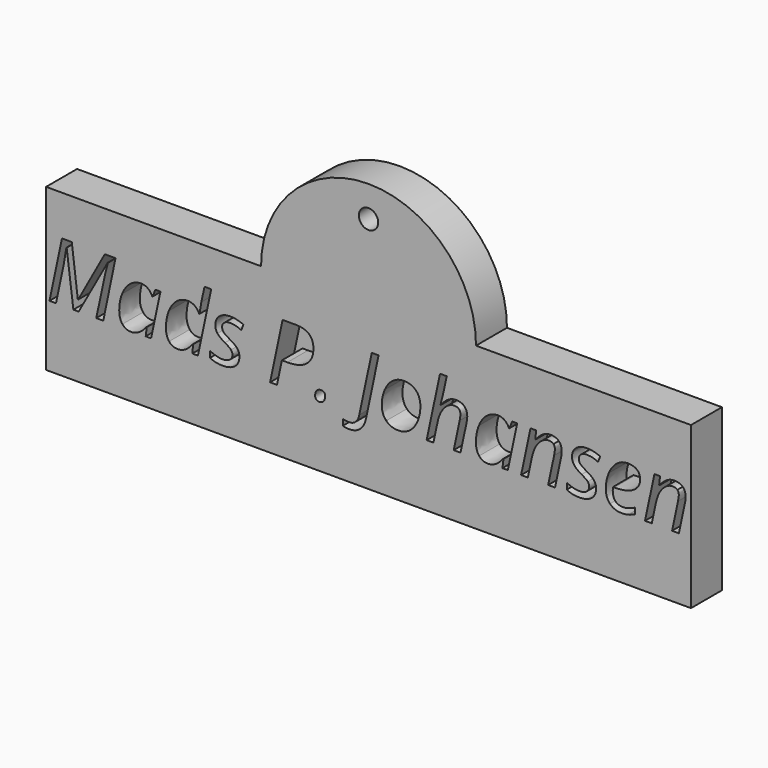
from build123d import *

# Parameters (mm, degrees)
F0_R     = 1.5
F1_DEPTH = 4
F2_R     = 1.5
F3_DEPTH = 2


with BuildPart() as f1:
    # F0 (on Front) → F1 (new body)
    with BuildSketch(Plane.XZ):
        Polygon((-16.667, 12.5), (-50, 12.5), (-50, -12.5), (50, -12.5), (50, 12.5), (16.667, 12.5), (0, 12.5), align=None)
        with BuildLine():
            add(Edge.make_bspline(
                [(-8.1103008935, -2.9097343631), (-8.2795785088, -2.746466604), (-8.2795785088, -2.4279442273)],
                knots=[0, 0, 0, 1, 1, 1], degree=2))
            add(Edge.make_bspline(
                [(-8.2795785088, -2.4279442273), (-8.2795785088, -1.9451524488), (-8.0251612645, -1.6606859237)],
                knots=[0, 0, 0, 1, 1, 1], degree=2))
            add(Edge.make_bspline(
                [(-8.0251612645, -1.6606859237), (-7.7707440202, -1.3762193986), (-7.3280179494, -1.3762193986)],
                knots=[0, 0, 0, 1, 1, 1], degree=2))
            add(Edge.make_bspline(
                [(-7.3280179494, -1.3762193986), (-7.0575744221, -1.3762193986), (-6.8923033775, -1.538485515)],
                knots=[0, 0, 0, 1, 1, 1], degree=2))
            add(Edge.make_bspline(
                [(-6.8923033775, -1.538485515), (-6.727032333, -1.7007516314), (-6.727032333, -2.0332970059)],
                knots=[0, 0, 0, 1, 1, 1], degree=2))
            add(Edge.make_bspline(
                [(-6.727032333, -2.0332970059), (-6.727032333, -2.478026362), (-6.9774430065, -2.7755142421)],
                knots=[0, 0, 0, 1, 1, 1], degree=2))
            add(Edge.make_bspline(
                [(-6.9774430065, -2.7755142421), (-7.22785368, -3.0730021222), (-7.6525501823, -3.0730021222)],
                knots=[0, 0, 0, 1, 1, 1], degree=2))
            add(Edge.make_bspline(
                [(-7.6525501823, -3.0730021222), (-7.9410232782, -3.0730021222), (-8.1103008935, -2.9097343631)],
                knots=[0, 0, 0, 1, 1, 1], degree=2))
        make_face(mode=Mode.SUBTRACT)
        with BuildLine():
            Line((-44.9477142514, -2.8907031519), (-45.7670579751, -2.8907031519))
            Line((-45.7670579751, -2.8907031519), (-46.8067630915, 5.2226026696))
            Line((-46.8067630915, 5.2226026696), (-46.8568452262, 5.2226026696))
            add(Edge.make_bspline(
                [(-46.8568452262, 5.2226026696), (-46.9009175047, 4.7718634573), (-47.0351376257, 3.9865755852)],
                knots=[0, 0, 0, 1, 1, 1], degree=2))
            add(Edge.make_bspline(
                [(-47.0351376257, 3.9865755852), (-47.1693577467, 3.2012877131), (-47.2695220161, 2.7365255031)],
                knots=[0, 0, 0, 1, 1, 1], degree=2))
            Line((-47.2695220161, 2.7365255031), (-48.4594735366, -2.8907031519))
            Line((-48.4594735366, -2.8907031519), (-49.4731359429, -2.8907031519))
            Line((-49.4731359429, -2.8907031519), (-47.5399655435, 6.262307786))
            Line((-47.5399655435, 6.262307786), (-46.0114587924, 6.262307786))
            Line((-46.0114587924, 6.262307786), (-45.079931087, -1.2760551292))
            Line((-45.079931087, -1.2760551292), (-45.0238390961, -1.2760551292))
            Line((-45.0238390961, -1.2760551292), (-40.8970711968, 6.262307786))
            Line((-40.8970711968, 6.262307786), (-39.2323410393, 6.262307786))
            Line((-39.2323410393, 6.262307786), (-41.1294523018, -2.8907031519))
            Line((-41.1294523018, -2.8907031519), (-42.2192395529, -2.8907031519))
            add(Edge.make_bspline(
                [(-42.2192395529, -2.8907031519), (-41.42994511, 0.8033551036), (-41.0102568212, 2.7785944962)],
                knots=[0, 0, 0, 1, 1, 1], degree=2))
            add(Edge.make_bspline(
                [(-41.0102568212, 2.7785944962), (-40.5905685324, 4.7538338888), (-40.4222925598, 5.2346223819)],
                knots=[0, 0, 0, 1, 1, 1], degree=2))
            Line((-40.4222925598, 5.2346223819), (-40.4583516968, 5.2346223819))
            Line((-40.4583516968, 5.2346223819), (-44.9477142514, -2.8907031519))
        make_face(mode=Mode.SUBTRACT)
        with BuildLine():
            add(Edge.make_bspline(
                [(-36.9856564766, 3.4637180989), (-36.2033735326, 4.0967562815), (-35.2698425418, 4.0967562815)],
                knots=[0, 0, 0, 1, 1, 1], degree=2))
            add(Edge.make_bspline(
                [(-35.2698425418, 4.0967562815), (-34.6948996354, 4.0967562815), (-34.2441604231, 3.7862470464)],
                knots=[0, 0, 0, 1, 1, 1], degree=2))
            add(Edge.make_bspline(
                [(-34.2441604231, 3.7862470464), (-33.7934212108, 3.4757378112), (-33.5430105373, 2.8947850487)],
                knots=[0, 0, 0, 1, 1, 1], degree=2))
            Line((-33.5430105373, 2.8947850487), (-33.4728955487, 2.8947850487))
            Line((-33.4728955487, 2.8947850487), (-33.0542089026, 3.9705493021))
            Line((-33.0542089026, 3.9705493021), (-32.2589046035, 3.9705493021))
            Line((-32.2589046035, 3.9705493021), (-33.717296366, -2.8907031519))
            Line((-33.717296366, -2.8907031519), (-34.5506630875, -2.8907031519))
            Line((-34.5506630875, -2.8907031519), (-34.3863936856, -1.5825577935))
            Line((-34.3863936856, -1.5825577935), (-34.4364758203, -1.5825577935))
            add(Edge.make_bspline(
                [(-34.4364758203, -1.5825577935), (-35.5583156376, -3.0169101314), (-36.7983492928, -3.0169101314)],
                knots=[0, 0, 0, 1, 1, 1], degree=2))
            add(Edge.make_bspline(
                [(-36.7983492928, -3.0169101314), (-37.6677751512, -3.0169101314), (-38.1625866421, -2.3968933038)],
                knots=[0, 0, 0, 1, 1, 1], degree=2))
            add(Edge.make_bspline(
                [(-38.1625866421, -2.3968933038), (-38.6573981329, -1.7768764762), (-38.6573981329, -0.6991089374)],
                knots=[0, 0, 0, 1, 1, 1], degree=2))
            add(Edge.make_bspline(
                [(-38.6573981329, -0.6991089374), (-38.6573981329, 0.6030265648), (-38.2126687768, 1.7168532405)],
                knots=[0, 0, 0, 1, 1, 1], degree=2))
            add(Edge.make_bspline(
                [(-38.2126687768, 1.7168532405), (-37.7679394206, 2.8306799163), (-36.9856564766, 3.4637180989)],
                knots=[0, 0, 0, 1, 1, 1], degree=2))
        make_face(mode=Mode.SUBTRACT)
        with BuildLine():
            add(Edge.make_bspline(
                [(-29.7447814416, 3.4757378112), (-28.9775231379, 4.0827332838), (-28.0259625786, 4.0827332838)],
                knots=[0, 0, 0, 1, 1, 1], degree=2))
            add(Edge.make_bspline(
                [(-28.0259625786, 4.0827332838), (-26.8119716335, 4.0827332838), (-26.2670780079, 2.8947850487)],
                knots=[0, 0, 0, 1, 1, 1], degree=2))
            Line((-26.2670780079, 2.8947850487), (-26.2049761609, 2.8947850487))
            add(Edge.make_bspline(
                [(-26.2049761609, 2.8947850487), (-26.0988020353, 3.8643751765), (-25.9225129212, 4.6095973409)],
                knots=[0, 0, 0, 1, 1, 1], degree=2))
            Line((-25.9225129212, 4.6095973409), (-25.4337112865, 6.8512736901))
            Line((-25.4337112865, 6.8512736901), (-24.3960094555, 6.8512736901))
            Line((-24.3960094555, 6.8512736901), (-26.4613966906, -2.8907031519))
            Line((-26.4613966906, -2.8907031519), (-27.330822549, -2.8907031519))
            Line((-27.330822549, -2.8907031519), (-27.1925958572, -1.5825577935))
            Line((-27.1925958572, -1.5825577935), (-27.2426779919, -1.5825577935))
            add(Edge.make_bspline(
                [(-27.2426779919, -1.5825577935), (-27.8757161745, -2.3638390949), (-28.4266196562, -2.6903746131)],
                knots=[0, 0, 0, 1, 1, 1], degree=2))
            add(Edge.make_bspline(
                [(-28.4266196562, -2.6903746131), (-28.9775231379, -3.0169101314), (-29.566489042, -3.0169101314)],
                knots=[0, 0, 0, 1, 1, 1], degree=2))
            add(Edge.make_bspline(
                [(-29.566489042, -3.0169101314), (-30.4359149004, -3.0169101314), (-30.9247165351, -2.4029031599)],
                knots=[0, 0, 0, 1, 1, 1], degree=2))
            add(Edge.make_bspline(
                [(-30.9247165351, -2.4029031599), (-31.4135181698, -1.7888961885), (-31.4135181698, -0.6991089374)],
                knots=[0, 0, 0, 1, 1, 1], degree=2))
            add(Edge.make_bspline(
                [(-31.4135181698, -0.6991089374), (-31.4135181698, 0.6410889872), (-30.9627789575, 1.7549156629)],
                knots=[0, 0, 0, 1, 1, 1], degree=2))
            add(Edge.make_bspline(
                [(-30.9627789575, 1.7549156629), (-30.5120397452, 2.8687423387), (-29.7447814416, 3.4757378112)],
                knots=[0, 0, 0, 1, 1, 1], degree=2))
        make_face(mode=Mode.SUBTRACT)
        with BuildLine():
            add(Edge.make_bspline(
                [(-20.1690772868, -0.245364797), (-20.0248407388, -0.5548723895), (-20.0248407388, -0.9435097548)],
                knots=[0, 0, 0, 1, 1, 1], degree=2))
            add(Edge.make_bspline(
                [(-20.0248407388, -0.9435097548), (-20.0248407388, -1.9211130241), (-20.7169758404, -2.4690115778)],
                knots=[0, 0, 0, 1, 1, 1], degree=2))
            add(Edge.make_bspline(
                [(-20.7169758404, -2.4690115778), (-21.4091109419, -3.0169101314), (-22.6671741656, -3.0169101314)],
                knots=[0, 0, 0, 1, 1, 1], degree=2))
            add(Edge.make_bspline(
                [(-22.6671741656, -3.0169101314), (-23.7249088505, -3.0169101314), (-24.5763051404, -2.5842004876)],
                knots=[0, 0, 0, 1, 1, 1], degree=2))
            Line((-24.5763051404, -2.5842004876), (-24.5763051404, -1.5945775059))
            add(Edge.make_bspline(
                [(-24.5763051404, -1.5945775059), (-24.1375856405, -1.8570078917), (-23.6307544373, -2.0012444396)],
                knots=[0, 0, 0, 1, 1, 1], degree=2))
            add(Edge.make_bspline(
                [(-23.6307544373, -2.0012444396), (-23.1239232341, -2.1454809876), (-22.6912135903, -2.1454809876)],
                knots=[0, 0, 0, 1, 1, 1], degree=2))
            add(Edge.make_bspline(
                [(-22.6912135903, -2.1454809876), (-21.9039224328, -2.1454809876), (-21.5032653552, -1.8329684671)],
                knots=[0, 0, 0, 1, 1, 1], degree=2))
            add(Edge.make_bspline(
                [(-21.5032653552, -1.8329684671), (-21.1026082776, -1.5204559465), (-21.1026082776, -1.0316543118)],
                knots=[0, 0, 0, 1, 1, 1], degree=2))
            add(Edge.make_bspline(
                [(-21.1026082776, -1.0316543118), (-21.1026082776, -0.6750695128), (-21.3209663849, -0.4306686954)],
                knots=[0, 0, 0, 1, 1, 1], degree=2))
            add(Edge.make_bspline(
                [(-21.3209663849, -0.4306686954), (-21.5393244922, -0.1862678781), (-22.266517088, 0.2404319096)],
                knots=[0, 0, 0, 1, 1, 1], degree=2))
            add(Edge.make_bspline(
                [(-22.266517088, 0.2404319096), (-23.0798509556, 0.697180978), (-23.4184061861, 1.1348988353)],
                knots=[0, 0, 0, 1, 1, 1], degree=2))
            add(Edge.make_bspline(
                [(-23.4184061861, 1.1348988353), (-23.7569614167, 1.5726166926), (-23.7569614167, 2.173602309)],
                knots=[0, 0, 0, 1, 1, 1], degree=2))
            add(Edge.make_bspline(
                [(-23.7569614167, 2.173602309), (-23.7569614167, 3.0370183113), (-23.1239232341, 3.5668872964)],
                knots=[0, 0, 0, 1, 1, 1], degree=2))
            add(Edge.make_bspline(
                [(-23.1239232341, 3.5668872964), (-22.4908850515, 4.0967562815), (-21.4591930766, 4.0967562815)],
                knots=[0, 0, 0, 1, 1, 1], degree=2))
            add(Edge.make_bspline(
                [(-21.4591930766, 4.0967562815), (-20.387435394, 4.0967562815), (-19.3918025562, 3.6319940715)],
                knots=[0, 0, 0, 1, 1, 1], degree=2))
            Line((-19.3918025562, 3.6319940715), (-19.7303577868, 2.7745879254))
            Line((-19.7303577868, 2.7745879254), (-20.0809327297, 2.9308441857))
            add(Edge.make_bspline(
                [(-20.0809327297, 2.9308441857), (-20.7139709123, 3.2012877131), (-21.4591930766, 3.2012877131)],
                knots=[0, 0, 0, 1, 1, 1], degree=2))
            add(Edge.make_bspline(
                [(-21.4591930766, 3.2012877131), (-22.0401458392, 3.2012877131), (-22.3726912136, 2.9288409003)],
                knots=[0, 0, 0, 1, 1, 1], degree=2))
            add(Edge.make_bspline(
                [(-22.3726912136, 2.9288409003), (-22.705236588, 2.6563940875), (-22.705236588, 2.2236844437)],
                knots=[0, 0, 0, 1, 1, 1], degree=2))
            add(Edge.make_bspline(
                [(-22.705236588, 2.2236844437), (-22.705236588, 1.8731095008), (-22.4828719099, 1.6226988273)],
                knots=[0, 0, 0, 1, 1, 1], degree=2))
            add(Edge.make_bspline(
                [(-22.4828719099, 1.6226988273), (-22.2605072319, 1.3722881538), (-21.5653672022, 0.9776409324)],
                knots=[0, 0, 0, 1, 1, 1], degree=2))
            add(Edge.make_bspline(
                [(-21.5653672022, 0.9776409324), (-20.8942665972, 0.6030265648), (-20.603790216, 0.3335846801)],
                knots=[0, 0, 0, 1, 1, 1], degree=2))
            add(Edge.make_bspline(
                [(-20.603790216, 0.3335846801), (-20.3133138347, 0.0641427954), (-20.1690772868, -0.245364797)],
                knots=[0, 0, 0, 1, 1, 1], degree=2))
        make_face(mode=Mode.SUBTRACT)
        with BuildLine():
            add(Edge.make_bspline(
                [(-0.3706077968, -2.9287655743), (-0.8654192876, -5.3006554737), (-3.0129412236, -5.3006554737)],
                knots=[0, 0, 0, 1, 1, 1], degree=2))
            add(Edge.make_bspline(
                [(-3.0129412236, -5.3006554737), (-3.6700188309, -5.3006554737), (-3.9705116391, -5.1443992135)],
                knots=[0, 0, 0, 1, 1, 1], degree=2))
            Line((-3.9705116391, -5.1443992135), (-3.9324492167, -4.2248912204))
            add(Edge.make_bspline(
                [(-3.9324492167, -4.2248912204), (-3.5017428583, -4.3490949144), (-3.0249609359, -4.3490949144)],
                knots=[0, 0, 0, 1, 1, 1], degree=2))
            add(Edge.make_bspline(
                [(-3.0249609359, -4.3490949144), (-2.3999358949, -4.3490949144), (-1.9892623903, -3.9584542638)],
                knots=[0, 0, 0, 1, 1, 1], degree=2))
            add(Edge.make_bspline(
                [(-1.9892623903, -3.9584542638), (-1.5785888858, -3.5678136131), (-1.4223326255, -2.8145783072)],
                knots=[0, 0, 0, 1, 1, 1], degree=2))
            Line((-1.4223326255, -2.8145783072), (0.4988180616, 6.262307786))
            Line((0.4988180616, 6.262307786), (1.5645658881, 6.262307786))
            Line((1.5645658881, 6.262307786), (-0.3706077968, -2.9287655743))
        make_face(mode=Mode.SUBTRACT)
        with BuildLine():
            add(Edge.make_bspline(
                [(-9.2371489242, 5.6703369538), (-8.5480187508, 5.0783661217), (-8.5480187508, 3.9024375989)],
                knots=[0, 0, 0, 1, 1, 1], degree=2))
            add(Edge.make_bspline(
                [(-8.5480187508, 3.9024375989), (-8.5480187508, 2.3498914232), (-9.5747025121, 1.5295460568)],
                knots=[0, 0, 0, 1, 1, 1], degree=2))
            add(Edge.make_bspline(
                [(-9.5747025121, 1.5295460568), (-10.6013862735, 0.7092006904), (-12.586642093, 0.7092006904)],
                knots=[0, 0, 0, 1, 1, 1], degree=2))
            Line((-12.586642093, 0.7092006904), (-13.4320285268, 0.7092006904))
            Line((-13.4320285268, 0.7092006904), (-14.2012901158, -2.8907031519))
            Line((-14.2012901158, -2.8907031519), (-15.2650346568, -2.8907031519))
            Line((-15.2650346568, -2.8907031519), (-13.3318642574, 6.262307786))
            Line((-13.3318642574, 6.262307786), (-11.2644737369, 6.262307786))
            add(Edge.make_bspline(
                [(-11.2644737369, 6.262307786), (-9.9262790977, 6.262307786), (-9.2371489242, 5.6703369538)],
                knots=[0, 0, 0, 1, 1, 1], degree=2))
        make_face(mode=Mode.SUBTRACT)
        with BuildLine():
            add(Edge.make_bspline(
                [(3.7551584599, 3.4977739505), (4.5314315477, 4.0586938592), (5.4749789655, 4.0586938592)],
                knots=[0, 0, 0, 1, 1, 1], degree=2))
            add(Edge.make_bspline(
                [(5.4749789655, 4.0586938592), (6.664930486, 4.0586938592), (7.3540606595, 3.3545390453)],
                knots=[0, 0, 0, 1, 1, 1], degree=2))
            add(Edge.make_bspline(
                [(7.3540606595, 3.3545390453), (8.043190833, 2.6503842314), (8.043190833, 1.4163604323)],
                knots=[0, 0, 0, 1, 1, 1], degree=2))
            add(Edge.make_bspline(
                [(8.043190833, 1.4163604323), (8.043190833, 0.2404319096), (7.5924516207, -0.805283063)],
                knots=[0, 0, 0, 1, 1, 1], degree=2))
            add(Edge.make_bspline(
                [(7.5924516207, -0.805283063), (7.1417124083, -1.8509980355), (6.3714491766, -2.4209327284)],
                knots=[0, 0, 0, 1, 1, 1], degree=2))
            add(Edge.make_bspline(
                [(6.3714491766, -2.4209327284), (5.6011859449, -2.9908674213), (4.6315958171, -2.9908674213)],
                knots=[0, 0, 0, 1, 1, 1], degree=2))
            add(Edge.make_bspline(
                [(4.6315958171, -2.9908674213), (3.4296245843, -2.9908674213), (2.746504267, -2.2837076794)],
                knots=[0, 0, 0, 1, 1, 1], degree=2))
            add(Edge.make_bspline(
                [(2.746504267, -2.2837076794), (2.0633839497, -1.5765479374), (2.0633839497, -0.3485339945)],
                knots=[0, 0, 0, 1, 1, 1], degree=2))
            add(Edge.make_bspline(
                [(2.0633839497, -0.3485339945), (2.0633839497, 0.841417526), (2.5211346608, 1.8891357839)],
                knots=[0, 0, 0, 1, 1, 1], degree=2))
            add(Edge.make_bspline(
                [(2.5211346608, 1.8891357839), (2.978885372, 2.9368540419), (3.7551584599, 3.4977739505)],
                knots=[0, 0, 0, 1, 1, 1], degree=2))
        make_face(mode=Mode.SUBTRACT)
        with BuildLine():
            Line((14.259385392, -2.8907031519), (13.2076605633, -2.8907031519))
            Line((13.2076605633, -2.8907031519), (14.135181698, 1.4424031424))
            add(Edge.make_bspline(
                [(14.135181698, 1.4424031424), (14.2473656797, 2.0293657611), (14.2473656797, 2.2857862908)],
                knots=[0, 0, 0, 1, 1, 1], degree=2))
            add(Edge.make_bspline(
                [(14.2473656797, 2.2857862908), (14.2473656797, 3.2133074254), (13.3278576866, 3.2133074254)],
                knots=[0, 0, 0, 1, 1, 1], degree=2))
            add(Edge.make_bspline(
                [(13.3278576866, 3.2133074254), (12.7689410633, 3.2133074254), (12.2400737209, 2.8437012713)],
                knots=[0, 0, 0, 1, 1, 1], degree=2))
            add(Edge.make_bspline(
                [(12.2400737209, 2.8437012713), (11.7112063785, 2.4740951172), (11.3075443728, 1.7699403033)],
                knots=[0, 0, 0, 1, 1, 1], degree=2))
            add(Edge.make_bspline(
                [(11.3075443728, 1.7699403033), (10.9038823671, 1.0657854894), (10.6975439721, 0.0701526516)],
                knots=[0, 0, 0, 1, 1, 1], degree=2))
            Line((10.6975439721, 0.0701526516), (10.0645057895, -2.8907031519))
            Line((10.0645057895, -2.8907031519), (9.0127809608, -2.8907031519))
            Line((9.0127809608, -2.8907031519), (11.0801714812, 6.8512736901))
            Line((11.0801714812, 6.8512736901), (12.1318963099, 6.8512736901))
            add(Edge.make_bspline(
                [(12.1318963099, 6.8512736901), (12.0177090428, 6.3364293454), (11.9145398453, 5.8546392095)],
                knots=[0, 0, 0, 1, 1, 1], degree=2))
            add(Edge.make_bspline(
                [(11.9145398453, 5.8546392095), (11.8113706479, 5.3728490737), (11.7021915942, 4.8750326548)],
                knots=[0, 0, 0, 1, 1, 1], degree=2))
            add(Edge.make_bspline(
                [(11.7021915942, 4.8750326548), (11.5930125406, 4.3772162359), (11.4648022757, 3.8323226103)],
                knots=[0, 0, 0, 1, 1, 1], degree=2))
            add(Edge.make_bspline(
                [(11.4648022757, 3.8323226103), (11.3365920109, 3.2874289848), (11.1663127529, 2.6503842314)],
                knots=[0, 0, 0, 1, 1, 1], degree=2))
            Line((11.1663127529, 2.6503842314), (11.2364277415, 2.6503842314))
            add(Edge.make_bspline(
                [(11.2364277415, 2.6503842314), (11.8253936456, 3.4196458204), (12.3973316239, 3.7511895521)],
                knots=[0, 0, 0, 1, 1, 1], degree=2))
            add(Edge.make_bspline(
                [(12.3973316239, 3.7511895521), (12.9692696021, 4.0827332838), (13.5962979286, 4.0827332838)],
                knots=[0, 0, 0, 1, 1, 1], degree=2))
            add(Edge.make_bspline(
                [(13.5962979286, 4.0827332838), (14.4156416523, 4.0827332838), (14.8633759365, 3.6319940715)],
                knots=[0, 0, 0, 1, 1, 1], degree=2))
            add(Edge.make_bspline(
                [(14.8633759365, 3.6319940715), (15.3111102208, 3.1812548592), (15.3111102208, 2.3559012793)],
                knots=[0, 0, 0, 1, 1, 1], degree=2))
            add(Edge.make_bspline(
                [(15.3111102208, 2.3559012793), (15.3111102208, 1.9672639141), (15.1668736728, 1.3161961629)],
                knots=[0, 0, 0, 1, 1, 1], degree=2))
            add(Edge.make_bspline(
                [(15.1668736728, 1.3161961629), (14.9224728555, 0.108215074), (14.259385392, -2.8907031519)],
                knots=[0, 0, 0, 1, 1, 1], degree=2))
        make_face(mode=Mode.SUBTRACT)
        with BuildLine():
            add(Edge.make_bspline(
                [(18.3290596578, 3.4637180989), (19.1113426019, 4.0967562815), (20.0448735927, 4.0967562815)],
                knots=[0, 0, 0, 1, 1, 1], degree=2))
            add(Edge.make_bspline(
                [(20.0448735927, 4.0967562815), (20.6198164991, 4.0967562815), (21.0705557114, 3.7862470464)],
                knots=[0, 0, 0, 1, 1, 1], degree=2))
            add(Edge.make_bspline(
                [(21.0705557114, 3.7862470464), (21.5212949237, 3.4757378112), (21.7717055972, 2.8947850487)],
                knots=[0, 0, 0, 1, 1, 1], degree=2))
            Line((21.7717055972, 2.8947850487), (21.8418205858, 2.8947850487))
            Line((21.8418205858, 2.8947850487), (22.2605072319, 3.9705493021))
            Line((22.2605072319, 3.9705493021), (23.0558115309, 3.9705493021))
            Line((23.0558115309, 3.9705493021), (21.5974197684, -2.8907031519))
            Line((21.5974197684, -2.8907031519), (20.764053047, -2.8907031519))
            Line((20.764053047, -2.8907031519), (20.9283224488, -1.5825577935))
            Line((20.9283224488, -1.5825577935), (20.8782403141, -1.5825577935))
            add(Edge.make_bspline(
                [(20.8782403141, -1.5825577935), (19.7564004968, -3.0169101314), (18.5163668416, -3.0169101314)],
                knots=[0, 0, 0, 1, 1, 1], degree=2))
            add(Edge.make_bspline(
                [(18.5163668416, -3.0169101314), (17.6469409832, -3.0169101314), (17.1521294924, -2.3968933038)],
                knots=[0, 0, 0, 1, 1, 1], degree=2))
            add(Edge.make_bspline(
                [(17.1521294924, -2.3968933038), (16.6573180015, -1.7768764762), (16.6573180015, -0.6991089374)],
                knots=[0, 0, 0, 1, 1, 1], degree=2))
            add(Edge.make_bspline(
                [(16.6573180015, -0.6991089374), (16.6573180015, 0.6030265648), (17.1020473577, 1.7168532405)],
                knots=[0, 0, 0, 1, 1, 1], degree=2))
            add(Edge.make_bspline(
                [(17.1020473577, 1.7168532405), (17.5467767138, 2.8306799163), (18.3290596578, 3.4637180989)],
                knots=[0, 0, 0, 1, 1, 1], degree=2))
        make_face(mode=Mode.SUBTRACT)
        with BuildLine():
            Line((28.9154212909, -2.8907031519), (27.8516767499, -2.8907031519))
            Line((27.8516767499, -2.8907031519), (28.7791978845, 1.4424031424))
            add(Edge.make_bspline(
                [(28.7791978845, 1.4424031424), (28.9034015786, 2.0934708935), (28.9034015786, 2.343881567)],
                knots=[0, 0, 0, 1, 1, 1], degree=2))
            add(Edge.make_bspline(
                [(28.9034015786, 2.343881567), (28.9034015786, 2.7365255031), (28.6810369005, 2.9749164642)],
                knots=[0, 0, 0, 1, 1, 1], degree=2))
            add(Edge.make_bspline(
                [(28.6810369005, 2.9749164642), (28.4586722224, 3.2133074254), (27.9718738732, 3.2133074254)],
                knots=[0, 0, 0, 1, 1, 1], degree=2))
            add(Edge.make_bspline(
                [(27.9718738732, 3.2133074254), (27.4129572499, 3.2133074254), (26.8840899074, 2.8376914152)],
                knots=[0, 0, 0, 1, 1, 1], degree=2))
            add(Edge.make_bspline(
                [(26.8840899074, 2.8376914152), (26.355222565, 2.4620754049), (25.9515605593, 1.7669353753)],
                knots=[0, 0, 0, 1, 1, 1], degree=2))
            add(Edge.make_bspline(
                [(25.9515605593, 1.7669353753), (25.5478985536, 1.0717953456), (25.3415601587, 0.0821723639)],
                knots=[0, 0, 0, 1, 1, 1], degree=2))
            Line((25.3415601587, 0.0821723639), (24.708521976, -2.8907031519))
            Line((24.708521976, -2.8907031519), (23.6567971473, -2.8907031519))
            Line((23.6567971473, -2.8907031519), (25.1232020514, 3.9705493021))
            Line((25.1232020514, 3.9705493021), (25.9926279098, 3.9705493021))
            Line((25.9926279098, 3.9705493021), (25.854401218, 2.7004663661))
            Line((25.854401218, 2.7004663661), (25.9185063504, 2.7004663661))
            add(Edge.make_bspline(
                [(25.9185063504, 2.7004663661), (26.5194919668, 3.4637180989), (27.0794102328, 3.7802371902)],
                knots=[0, 0, 0, 1, 1, 1], degree=2))
            add(Edge.make_bspline(
                [(27.0794102328, 3.7802371902), (27.6393284987, 4.0967562815), (28.2403141151, 4.0967562815)],
                knots=[0, 0, 0, 1, 1, 1], degree=2))
            add(Edge.make_bspline(
                [(28.2403141151, 4.0967562815), (29.0356184142, 4.0967562815), (29.4953724108, 3.6610417096)],
                knots=[0, 0, 0, 1, 1, 1], degree=2))
            add(Edge.make_bspline(
                [(29.4953724108, 3.6610417096), (29.9551264073, 3.2253271377), (29.9551264073, 2.4440458364)],
                knots=[0, 0, 0, 1, 1, 1], degree=2))
            add(Edge.make_bspline(
                [(29.9551264073, 2.4440458364), (29.9551264073, 1.9492343456), (29.8108898594, 1.3161961629)],
                knots=[0, 0, 0, 1, 1, 1], degree=2))
            Line((29.8108898594, 1.3161961629), (28.9154212909, -2.8907031519))
        make_face(mode=Mode.SUBTRACT)
        with BuildLine():
            add(Edge.make_bspline(
                [(35.1456388477, -0.245364797), (35.2898753956, -0.5548723895), (35.2898753956, -0.9435097548)],
                knots=[0, 0, 0, 1, 1, 1], degree=2))
            add(Edge.make_bspline(
                [(35.2898753956, -0.9435097548), (35.2898753956, -1.9211130241), (34.5977402941, -2.4690115778)],
                knots=[0, 0, 0, 1, 1, 1], degree=2))
            add(Edge.make_bspline(
                [(34.5977402941, -2.4690115778), (33.9056051925, -3.0169101314), (32.6475419688, -3.0169101314)],
                knots=[0, 0, 0, 1, 1, 1], degree=2))
            add(Edge.make_bspline(
                [(32.6475419688, -3.0169101314), (31.5898072839, -3.0169101314), (30.738410994, -2.5842004876)],
                knots=[0, 0, 0, 1, 1, 1], degree=2))
            Line((30.738410994, -2.5842004876), (30.738410994, -1.5945775059))
            add(Edge.make_bspline(
                [(30.738410994, -1.5945775059), (31.177130494, -1.8570078917), (31.6839616972, -2.0012444396)],
                knots=[0, 0, 0, 1, 1, 1], degree=2))
            add(Edge.make_bspline(
                [(31.6839616972, -2.0012444396), (32.1907929004, -2.1454809876), (32.6235025442, -2.1454809876)],
                knots=[0, 0, 0, 1, 1, 1], degree=2))
            add(Edge.make_bspline(
                [(32.6235025442, -2.1454809876), (33.4107937017, -2.1454809876), (33.8114507793, -1.8329684671)],
                knots=[0, 0, 0, 1, 1, 1], degree=2))
            add(Edge.make_bspline(
                [(33.8114507793, -1.8329684671), (34.2121078569, -1.5204559465), (34.2121078569, -1.0316543118)],
                knots=[0, 0, 0, 1, 1, 1], degree=2))
            add(Edge.make_bspline(
                [(34.2121078569, -1.0316543118), (34.2121078569, -0.6750695128), (33.9937497496, -0.4306686954)],
                knots=[0, 0, 0, 1, 1, 1], degree=2))
            add(Edge.make_bspline(
                [(33.9937497496, -0.4306686954), (33.7753916423, -0.1862678781), (33.0481990464, 0.2404319096)],
                knots=[0, 0, 0, 1, 1, 1], degree=2))
            add(Edge.make_bspline(
                [(33.0481990464, 0.2404319096), (32.2348651789, 0.697180978), (31.8963099483, 1.1348988353)],
                knots=[0, 0, 0, 1, 1, 1], degree=2))
            add(Edge.make_bspline(
                [(31.8963099483, 1.1348988353), (31.5577547177, 1.5726166926), (31.5577547177, 2.173602309)],
                knots=[0, 0, 0, 1, 1, 1], degree=2))
            add(Edge.make_bspline(
                [(31.5577547177, 2.173602309), (31.5577547177, 3.0370183113), (32.1907929004, 3.5668872964)],
                knots=[0, 0, 0, 1, 1, 1], degree=2))
            add(Edge.make_bspline(
                [(32.1907929004, 3.5668872964), (32.823831083, 4.0967562815), (33.8555230578, 4.0967562815)],
                knots=[0, 0, 0, 1, 1, 1], degree=2))
            add(Edge.make_bspline(
                [(33.8555230578, 4.0967562815), (34.9272807404, 4.0967562815), (35.9229135783, 3.6319940715)],
                knots=[0, 0, 0, 1, 1, 1], degree=2))
            Line((35.9229135783, 3.6319940715), (35.5843583477, 2.7745879254))
            Line((35.5843583477, 2.7745879254), (35.2337834048, 2.9308441857))
            add(Edge.make_bspline(
                [(35.2337834048, 2.9308441857), (34.6007452222, 3.2012877131), (33.8555230578, 3.2012877131)],
                knots=[0, 0, 0, 1, 1, 1], degree=2))
            add(Edge.make_bspline(
                [(33.8555230578, 3.2012877131), (33.2745702953, 3.2012877131), (32.9420249209, 2.9288409003)],
                knots=[0, 0, 0, 1, 1, 1], degree=2))
            add(Edge.make_bspline(
                [(32.9420249209, 2.9288409003), (32.6094795465, 2.6563940875), (32.6094795465, 2.2236844437)],
                knots=[0, 0, 0, 1, 1, 1], degree=2))
            add(Edge.make_bspline(
                [(32.6094795465, 2.2236844437), (32.6094795465, 1.8731095008), (32.8318442245, 1.6226988273)],
                knots=[0, 0, 0, 1, 1, 1], degree=2))
            add(Edge.make_bspline(
                [(32.8318442245, 1.6226988273), (33.0542089026, 1.3722881538), (33.7493489322, 0.9776409324)],
                knots=[0, 0, 0, 1, 1, 1], degree=2))
            add(Edge.make_bspline(
                [(33.7493489322, 0.9776409324), (34.4204495372, 0.6030265648), (34.7109259185, 0.3335846801)],
                knots=[0, 0, 0, 1, 1, 1], degree=2))
            add(Edge.make_bspline(
                [(34.7109259185, 0.3335846801), (35.0014022998, 0.0641427954), (35.1456388477, -0.245364797)],
                knots=[0, 0, 0, 1, 1, 1], degree=2))
        make_face(mode=Mode.SUBTRACT)
        with BuildLine():
            add(Edge.make_bspline(
                [(40.2540165872, -2.906729435), (39.8032773749, -3.0169101314), (39.2603870347, -3.0169101314)],
                knots=[0, 0, 0, 1, 1, 1], degree=2))
            add(Edge.make_bspline(
                [(39.2603870347, -3.0169101314), (38.1084979366, -3.0169101314), (37.4504186866, -2.3337898141)],
                knots=[0, 0, 0, 1, 1, 1], degree=2))
            add(Edge.make_bspline(
                [(37.4504186866, -2.3337898141), (36.7923394367, -1.6506694967), (36.7923394367, -0.4426884078)],
                knots=[0, 0, 0, 1, 1, 1], degree=2))
            add(Edge.make_bspline(
                [(36.7923394367, -0.4426884078), (36.7923394367, 0.733240115), (37.2591049321, 1.8140125819)],
                knots=[0, 0, 0, 1, 1, 1], degree=2))
            add(Edge.make_bspline(
                [(37.2591049321, 1.8140125819), (37.7258704275, 2.8947850487), (38.4961336592, 3.4957706651)],
                knots=[0, 0, 0, 1, 1, 1], degree=2))
            add(Edge.make_bspline(
                [(38.4961336592, 3.4957706651), (39.2663968909, 4.0967562815), (40.1919147402, 4.0967562815)],
                knots=[0, 0, 0, 1, 1, 1], degree=2))
            add(Edge.make_bspline(
                [(40.1919147402, 4.0967562815), (41.1494851557, 4.0967562815), (41.6322769342, 3.6800729208)],
                knots=[0, 0, 0, 1, 1, 1], degree=2))
            add(Edge.make_bspline(
                [(41.6322769342, 3.6800729208), (42.1150687127, 3.2633895601), (42.1150687127, 2.5181673958)],
                knots=[0, 0, 0, 1, 1, 1], degree=2))
            add(Edge.make_bspline(
                [(42.1150687127, 2.5181673958), (42.1150687127, 1.3923210077), (41.0753635963, 0.7502680408)],
                knots=[0, 0, 0, 1, 1, 1], degree=2))
            add(Edge.make_bspline(
                [(41.0753635963, 0.7502680408), (40.0356584799, 0.108215074), (38.1004847951, 0.108215074)],
                knots=[0, 0, 0, 1, 1, 1], degree=2))
            Line((38.1004847951, 0.108215074), (37.8941464001, 0.108215074))
            Line((37.8941464001, 0.108215074), (37.8701069754, -0.3926062731))
            add(Edge.make_bspline(
                [(37.8701069754, -0.3926062731), (37.8701069754, -1.2119499968), (38.2547377699, -1.672705636)],
                knots=[0, 0, 0, 1, 1, 1], degree=2))
            add(Edge.make_bspline(
                [(38.2547377699, -1.672705636), (38.6393685644, -2.1334612753), (39.4466925758, -2.1334612753)],
                knots=[0, 0, 0, 1, 1, 1], degree=2))
            add(Edge.make_bspline(
                [(39.4466925758, -2.1334612753), (39.8413397973, -2.1334612753), (40.258023158, -2.0202756508)],
                knots=[0, 0, 0, 1, 1, 1], degree=2))
            add(Edge.make_bspline(
                [(40.258023158, -2.0202756508), (40.6747065187, -1.9070900264), (41.2937217036, -1.6065972182)],
                knots=[0, 0, 0, 1, 1, 1], degree=2))
            Line((41.2937217036, -1.6065972182), (41.2937217036, -2.5220986405))
            add(Edge.make_bspline(
                [(41.2937217036, -2.5220986405), (40.7047557995, -2.7965487387), (40.2540165872, -2.906729435)],
                knots=[0, 0, 0, 1, 1, 1], degree=2))
        make_face(mode=Mode.SUBTRACT)
        with BuildLine():
            Line((48.1289314476, -2.8907031519), (47.0651869065, -2.8907031519))
            Line((47.0651869065, -2.8907031519), (47.9927080412, 1.4424031424))
            add(Edge.make_bspline(
                [(47.9927080412, 1.4424031424), (48.1169117352, 2.0934708935), (48.1169117352, 2.343881567)],
                knots=[0, 0, 0, 1, 1, 1], degree=2))
            add(Edge.make_bspline(
                [(48.1169117352, 2.343881567), (48.1169117352, 2.7365255031), (47.8945470572, 2.9749164642)],
                knots=[0, 0, 0, 1, 1, 1], degree=2))
            add(Edge.make_bspline(
                [(47.8945470572, 2.9749164642), (47.6721823791, 3.2133074254), (47.1853840298, 3.2133074254)],
                knots=[0, 0, 0, 1, 1, 1], degree=2))
            add(Edge.make_bspline(
                [(47.1853840298, 3.2133074254), (46.6264674065, 3.2133074254), (46.0976000641, 2.8376914152)],
                knots=[0, 0, 0, 1, 1, 1], degree=2))
            add(Edge.make_bspline(
                [(46.0976000641, 2.8376914152), (45.5687327217, 2.4620754049), (45.165070716, 1.7669353753)],
                knots=[0, 0, 0, 1, 1, 1], degree=2))
            add(Edge.make_bspline(
                [(45.165070716, 1.7669353753), (44.7614087103, 1.0717953456), (44.5550703153, 0.0821723639)],
                knots=[0, 0, 0, 1, 1, 1], degree=2))
            Line((44.5550703153, 0.0821723639), (43.9220321327, -2.8907031519))
            Line((43.9220321327, -2.8907031519), (42.870307304, -2.8907031519))
            Line((42.870307304, -2.8907031519), (44.336712208, 3.9705493021))
            Line((44.336712208, 3.9705493021), (45.2061380664, 3.9705493021))
            Line((45.2061380664, 3.9705493021), (45.0679113747, 2.7004663661))
            Line((45.0679113747, 2.7004663661), (45.1320165071, 2.7004663661))
            add(Edge.make_bspline(
                [(45.1320165071, 2.7004663661), (45.7330021235, 3.4637180989), (46.2929203894, 3.7802371902)],
                knots=[0, 0, 0, 1, 1, 1], degree=2))
            add(Edge.make_bspline(
                [(46.2929203894, 3.7802371902), (46.8528386554, 4.0967562815), (47.4538242718, 4.0967562815)],
                knots=[0, 0, 0, 1, 1, 1], degree=2))
            add(Edge.make_bspline(
                [(47.4538242718, 4.0967562815), (48.2491285709, 4.0967562815), (48.7088825674, 3.6610417096)],
                knots=[0, 0, 0, 1, 1, 1], degree=2))
            add(Edge.make_bspline(
                [(48.7088825674, 3.6610417096), (49.168636564, 3.2253271377), (49.168636564, 2.4440458364)],
                knots=[0, 0, 0, 1, 1, 1], degree=2))
            add(Edge.make_bspline(
                [(49.168636564, 2.4440458364), (49.168636564, 1.9492343456), (49.024400016, 1.3161961629)],
                knots=[0, 0, 0, 1, 1, 1], degree=2))
            Line((49.024400016, 1.3161961629), (48.1289314476, -2.8907031519))
        make_face(mode=Mode.SUBTRACT)
        with BuildLine():
            ThreePointArc((16.667, 12.5), (0, 29.167), (-16.667, 12.5))
            Line((-16.667, 12.5), (0, 12.5))
            Line((0, 12.5), (16.667, 12.5))
        make_face()
        with Locations((0, 24.3615116924)):
            Circle(F0_R, mode=Mode.SUBTRACT)
    extrude(amount=F1_DEPTH)

    # F2 (on face) → F3 (join)
    with BuildSketch(Plane(origin=(0, 0, 0), x_dir=(-1, 0, 0), z_dir=(0, 1, 0))):
        with BuildLine():
            ThreePointArc((16.667, 12.5), (0, 29.167), (-16.667, 12.5))
            Line((-16.667, 12.5), (-50, 12.5))
            Line((-50, 12.5), (-50, -12.5))
            Line((-50, -12.5), (50, -12.5))
            Line((50, -12.5), (50, 12.5))
            Line((50, 12.5), (16.667, 12.5))
        make_face()
        with BuildLine():
            Line((-47.9927080412, 1.4424031424), (-47.0651869065, -2.8907031519))
            Line((-47.0651869065, -2.8907031519), (-48.1289314476, -2.8907031519))
            Line((-48.1289314476, -2.8907031519), (-49.024400016, 1.3161961629))
            add(Edge.make_bspline(
                [(-45.1320165071, 2.7004663661), (-45.7330021235, 3.4637180989), (-46.8528386554, 4.0967562815), (-48.2491285709, 4.0967562815), (-49.168636564, 3.2253271377), (-49.168636564, 1.9492343456), (-49.024400016, 1.3161961629)],
                knots=[0, 0, 0, 1, 2, 3.3233333333, 4.6466666667, 5.4847777778, 5.4847777778, 5.4847777778], degree=2))
            Line((-45.1320165071, 2.7004663661), (-45.0679113747, 2.7004663661))
            Line((-45.0679113747, 2.7004663661), (-45.2061380664, 3.9705493021))
            Line((-45.2061380664, 3.9705493021), (-44.336712208, 3.9705493021))
            Line((-44.336712208, 3.9705493021), (-42.870307304, -2.8907031519))
            Line((-42.870307304, -2.8907031519), (-43.9220321327, -2.8907031519))
            Line((-43.9220321327, -2.8907031519), (-44.5550703153, 0.0821723639))
            add(Edge.make_bspline(
                [(-47.9927080412, 1.4424031424), (-48.1169117352, 2.0934708935), (-48.1169117352, 2.7365255031), (-47.6721823791, 3.2133074254), (-46.6264674065, 3.2133074254), (-45.5687327217, 2.4620754049), (-44.7614087103, 1.0717953456), (-44.5550703153, 0.0821723639)],
                knots=[0, 0, 0, 1, 2.568, 4.136, 5.9362962963, 7.7365925926, 9.5368888889, 9.5368888889, 9.5368888889], degree=2))
        make_face(mode=Mode.SUBTRACT)
        with BuildLine():
            Line((-37.8701069754, -0.3926062731), (-37.8941464001, 0.108215074))
            Line((-37.8941464001, 0.108215074), (-38.1004847951, 0.108215074))
            add(Edge.make_bspline(
                [(-41.2937217036, -2.5220986405), (-40.7047557995, -2.7965487387), (-39.8032773749, -3.0169101314), (-38.1084979366, -3.0169101314), (-36.7923394367, -1.6506694967), (-36.7923394367, 0.733240115), (-37.7258704275, 2.8947850487), (-39.2663968909, 4.0967562815), (-41.1494851557, 4.0967562815), (-42.1150687127, 3.2633895601), (-42.1150687127, 1.3923210077), (-40.0356584799, 0.108215074), (-38.1004847951, 0.108215074)],
                knots=[0, 0, 0, 1, 2, 4.1217712177, 6.2435424354, 8.3090145827, 10.3744867299, 12.4399588772, 14.5769625274, 16.7139661776, 19.9424501868, 23.1709341959, 23.1709341959, 23.1709341959], degree=2))
            Line((-41.2937217036, -2.5220986405), (-41.2937217036, -1.6065972182))
            add(Edge.make_bspline(
                [(-37.8701069754, -0.3926062731), (-37.8701069754, -1.2119499968), (-38.6393685644, -2.1334612753), (-39.8413397973, -2.1334612753), (-40.6747065187, -1.9070900264), (-41.2937217036, -1.6065972182)],
                knots=[0, 0, 0, 1, 2, 2.4888337469, 2.9776674938, 2.9776674938, 2.9776674938], degree=2))
        make_face(mode=Mode.SUBTRACT)
        with BuildLine():
            add(Edge.make_bspline(
                [(-30.738410994, -1.5945775059), (-31.177130494, -1.8570078917), (-32.1907929004, -2.1454809876), (-33.4107937017, -2.1454809876), (-34.2121078569, -1.5204559465), (-34.2121078569, -0.6750695128), (-33.7753916423, -0.1862678781), (-33.0481990464, 0.2404319096)],
                knots=[0, 0, 0, 1, 2, 3.8194444444, 5.6388888889, 6.9661885246, 8.2934881603, 8.2934881603, 8.2934881603], degree=2))
            Line((-30.738410994, -1.5945775059), (-30.738410994, -2.5842004876))
            add(Edge.make_bspline(
                [(-33.7493489322, 0.9776409324), (-34.4204495372, 0.6030265648), (-35.0014022998, 0.0641427954), (-35.2898753956, -0.5548723895), (-35.2898753956, -1.9211130241), (-33.9056051925, -3.0169101314), (-31.5898072839, -3.0169101314), (-30.738410994, -2.5842004876)],
                knots=[0, 0, 0, 1, 2, 3, 5.5154639175, 8.0309278351, 10.1458401734, 10.1458401734, 10.1458401734], degree=2))
            add(Edge.make_bspline(
                [(-35.2337834048, 2.9308441857), (-34.6007452222, 3.2012877131), (-33.2745702953, 3.2012877131), (-32.6094795465, 2.6563940875), (-32.6094795465, 1.8731095008), (-33.0542089026, 1.3722881538), (-33.7493489322, 0.9776409324)],
                knots=[0, 0, 0, 1, 1.7795698925, 2.5591397849, 3.1907357626, 3.8223317403, 3.8223317403, 3.8223317403], degree=2))
            Line((-35.2337834048, 2.9308441857), (-35.5843583477, 2.7745879254))
            Line((-35.5843583477, 2.7745879254), (-35.9229135783, 3.6319940715))
            add(Edge.make_bspline(
                [(-33.0481990464, 0.2404319096), (-32.2348651789, 0.697180978), (-31.5577547177, 1.5726166926), (-31.5577547177, 3.0370183113), (-32.823831083, 4.0967562815), (-34.9272807404, 4.0967562815), (-35.9229135783, 3.6319940715)],
                knots=[0, 0, 0, 1, 2, 3.4366666667, 4.8733333333, 6.3657928803, 6.3657928803, 6.3657928803], degree=2))
        make_face(mode=Mode.SUBTRACT)
        with BuildLine():
            Line((-28.7791978845, 1.4424031424), (-27.8516767499, -2.8907031519))
            Line((-27.8516767499, -2.8907031519), (-28.9154212909, -2.8907031519))
            Line((-28.9154212909, -2.8907031519), (-29.8108898594, 1.3161961629))
            add(Edge.make_bspline(
                [(-25.9185063504, 2.7004663661), (-26.5194919668, 3.4637180989), (-27.6393284987, 4.0967562815), (-29.0356184142, 4.0967562815), (-29.9551264073, 3.2253271377), (-29.9551264073, 1.9492343456), (-29.8108898594, 1.3161961629)],
                knots=[0, 0, 0, 1, 2, 3.3233333333, 4.6466666667, 5.4847777778, 5.4847777778, 5.4847777778], degree=2))
            Line((-25.9185063504, 2.7004663661), (-25.854401218, 2.7004663661))
            Line((-25.854401218, 2.7004663661), (-25.9926279098, 3.9705493021))
            Line((-25.9926279098, 3.9705493021), (-25.1232020514, 3.9705493021))
            Line((-25.1232020514, 3.9705493021), (-23.6567971473, -2.8907031519))
            Line((-23.6567971473, -2.8907031519), (-24.708521976, -2.8907031519))
            Line((-24.708521976, -2.8907031519), (-25.3415601587, 0.0821723639))
            add(Edge.make_bspline(
                [(-28.7791978845, 1.4424031424), (-28.9034015786, 2.0934708935), (-28.9034015786, 2.7365255031), (-28.4586722224, 3.2133074254), (-27.4129572499, 3.2133074254), (-26.355222565, 2.4620754049), (-25.5478985536, 1.0717953456), (-25.3415601587, 0.0821723639)],
                knots=[0, 0, 0, 1, 2.568, 4.136, 5.9362962963, 7.7365925926, 9.5368888889, 9.5368888889, 9.5368888889], degree=2))
        make_face(mode=Mode.SUBTRACT)
        with BuildLine():
            Line((-22.2605072319, 3.9705493021), (-21.8418205858, 2.8947850487))
            Line((-21.8418205858, 2.8947850487), (-21.7717055972, 2.8947850487))
            add(Edge.make_bspline(
                [(-20.8782403141, -1.5825577935), (-19.7564004968, -3.0169101314), (-17.6469409832, -3.0169101314), (-16.6573180015, -1.7768764762), (-16.6573180015, 0.6030265648), (-17.5467767138, 2.8306799163), (-19.1113426019, 4.0967562815), (-20.6198164991, 4.0967562815), (-21.5212949237, 3.4757378112), (-21.7717055972, 2.8947850487)],
                knots=[0, 0, 0, 1, 1.7011308562, 2.4022617124, 3.2493528956, 4.0964440788, 4.9435352619, 5.4652416344, 5.9869480069, 5.9869480069, 5.9869480069], degree=2))
            Line((-20.8782403141, -1.5825577935), (-20.9283224488, -1.5825577935))
            Line((-20.9283224488, -1.5825577935), (-20.764053047, -2.8907031519))
            Line((-20.764053047, -2.8907031519), (-21.5974197684, -2.8907031519))
            Line((-21.5974197684, -2.8907031519), (-23.0558115309, 3.9705493021))
            Line((-23.0558115309, 3.9705493021), (-22.2605072319, 3.9705493021))
        make_face(mode=Mode.SUBTRACT)
        with BuildLine():
            Line((-14.135181698, 1.4424031424), (-13.2076605633, -2.8907031519))
            Line((-13.2076605633, -2.8907031519), (-14.259385392, -2.8907031519))
            add(Edge.make_bspline(
                [(-15.1668736728, 1.3161961629), (-14.9224728555, 0.108215074), (-14.259385392, -2.8907031519)],
                knots=[0, 0, 0, 1, 1, 1], degree=2))
            add(Edge.make_bspline(
                [(-11.2364277415, 2.6503842314), (-11.8253936456, 3.4196458204), (-12.9692696021, 4.0827332838), (-14.4156416523, 4.0827332838), (-15.3111102208, 3.1812548592), (-15.3111102208, 1.9672639141), (-15.1668736728, 1.3161961629)],
                knots=[0, 0, 0, 1, 2, 3.3067092652, 4.6134185304, 5.2287136698, 5.2287136698, 5.2287136698], degree=2))
            Line((-11.2364277415, 2.6503842314), (-11.1663127529, 2.6503842314))
            add(Edge.make_bspline(
                [(-12.1318963099, 6.8512736901), (-12.0177090428, 6.3364293454), (-11.8113706479, 5.3728490737), (-11.5930125406, 4.3772162359), (-11.3365920109, 3.2874289848), (-11.1663127529, 2.6503842314)],
                knots=[0, 0, 0, 1, 2, 3, 4, 4, 4], degree=2))
            Line((-12.1318963099, 6.8512736901), (-11.0801714812, 6.8512736901))
            Line((-11.0801714812, 6.8512736901), (-9.0127809608, -2.8907031519))
            Line((-9.0127809608, -2.8907031519), (-10.0645057895, -2.8907031519))
            Line((-10.0645057895, -2.8907031519), (-10.6975439721, 0.0701526516))
            add(Edge.make_bspline(
                [(-14.135181698, 1.4424031424), (-14.2473656797, 2.0293657611), (-14.2473656797, 3.2133074254), (-12.7689410633, 3.2133074254), (-11.7112063785, 2.4740951172), (-10.9038823671, 1.0657854894), (-10.6975439721, 0.0701526516)],
                knots=[0, 0, 0, 1, 4.6171875, 6.815870098, 9.0145526961, 11.2132352941, 11.2132352941, 11.2132352941], degree=2))
        make_face(mode=Mode.SUBTRACT)
        with BuildLine():
            add(Edge.make_bspline(
                [(-5.4749789655, 4.0586938592), (-6.664930486, 4.0586938592), (-8.043190833, 2.6503842314), (-8.043190833, 0.2404319096), (-7.1417124083, -1.8509980355), (-5.6011859449, -2.9908674213), (-3.4296245843, -2.9908674213), (-2.0633839497, -1.5765479374), (-2.0633839497, 0.841417526), (-2.978885372, 2.9368540419), (-4.5314315477, 4.0586938592), (-5.4749789655, 4.0586938592)],
                knots=[0, 0, 0, 1, 2, 2.9529220779, 3.9058441558, 4.8587662338, 6.0400745948, 7.2213829559, 8.366076539, 9.5107701222, 10.6554637053, 10.6554637053, 10.6554637053], degree=2))
        make_face(mode=Mode.SUBTRACT)
        with BuildLine():
            add(Edge.make_bspline(
                [(8.2795785088, -2.4279442273), (8.2795785088, -1.9451524488), (7.7707440202, -1.3762193986), (7.0575744221, -1.3762193986), (6.727032333, -1.7007516314), (6.727032333, -2.478026362), (7.22785368, -3.0730021222), (7.9410232782, -3.0730021222), (8.2795785088, -2.746466604), (8.2795785088, -2.4279442273)],
                knots=[0, 0, 0, 1, 2, 2.6108597285, 3.221719457, 4.0386523469, 4.8555852369, 5.4104830489, 5.9653808609, 5.9653808609, 5.9653808609], degree=2))
        make_face(mode=Mode.SUBTRACT)
        with BuildLine():
            add(Edge.make_bspline(
                [(0.3706077968, -2.9287655743), (0.8654192876, -5.3006554737), (3.6700188309, -5.3006554737), (3.9705116391, -5.1443992135)],
                knots=[0, 0, 0, 1, 1.3059701493, 1.3059701493, 1.3059701493], degree=2))
            Line((0.3706077968, -2.9287655743), (-1.5645658881, 6.262307786))
            Line((-1.5645658881, 6.262307786), (-0.4988180616, 6.262307786))
            Line((-0.4988180616, 6.262307786), (1.4223326255, -2.8145783072))
            add(Edge.make_bspline(
                [(3.9324492167, -4.2248912204), (3.5017428583, -4.3490949144), (2.3999358949, -4.3490949144), (1.5785888858, -3.5678136131), (1.4223326255, -2.8145783072)],
                knots=[0, 0, 0, 1, 2.3109243697, 3.6218487395, 3.6218487395, 3.6218487395], degree=2))
            Line((3.9324492167, -4.2248912204), (3.9705116391, -5.1443992135))
        make_face(mode=Mode.SUBTRACT)
        with BuildLine():
            Line((14.2012901158, -2.8907031519), (13.4320285268, 0.7092006904))
            Line((13.4320285268, 0.7092006904), (12.586642093, 0.7092006904))
            add(Edge.make_bspline(
                [(11.2644737369, 6.262307786), (9.9262790977, 6.262307786), (8.5480187508, 5.0783661217), (8.5480187508, 2.3498914232), (10.6013862735, 0.7092006904), (12.586642093, 0.7092006904)],
                knots=[0, 0, 0, 1, 2, 3.3202725724, 4.6405451448, 4.6405451448, 4.6405451448], degree=2))
            Line((11.2644737369, 6.262307786), (13.3318642574, 6.262307786))
            Line((13.3318642574, 6.262307786), (15.2650346568, -2.8907031519))
            Line((15.2650346568, -2.8907031519), (14.2012901158, -2.8907031519))
        make_face(mode=Mode.SUBTRACT)
        with BuildLine():
            add(Edge.make_bspline(
                [(24.5763051404, -1.5945775059), (24.1375856405, -1.8570078917), (23.1239232341, -2.1454809876), (21.9039224328, -2.1454809876), (21.1026082776, -1.5204559465), (21.1026082776, -0.6750695128), (21.5393244922, -0.1862678781), (22.266517088, 0.2404319096)],
                knots=[0, 0, 0, 1, 2, 3.8194444444, 5.6388888889, 6.9661885246, 8.2934881603, 8.2934881603, 8.2934881603], degree=2))
            Line((24.5763051404, -1.5945775059), (24.5763051404, -2.5842004876))
            add(Edge.make_bspline(
                [(21.5653672022, 0.9776409324), (20.8942665972, 0.6030265648), (20.3133138347, 0.0641427954), (20.0248407388, -0.5548723895), (20.0248407388, -1.9211130241), (21.4091109419, -3.0169101314), (23.7249088505, -3.0169101314), (24.5763051404, -2.5842004876)],
                knots=[0, 0, 0, 1, 2, 3, 5.5154639175, 8.0309278351, 10.1458401734, 10.1458401734, 10.1458401734], degree=2))
            add(Edge.make_bspline(
                [(20.0809327297, 2.9308441857), (20.7139709123, 3.2012877131), (22.0401458392, 3.2012877131), (22.705236588, 2.6563940875), (22.705236588, 1.8731095008), (22.2605072319, 1.3722881538), (21.5653672022, 0.9776409324)],
                knots=[0, 0, 0, 1, 1.7795698925, 2.5591397849, 3.1907357626, 3.8223317403, 3.8223317403, 3.8223317403], degree=2))
            Line((20.0809327297, 2.9308441857), (19.7303577868, 2.7745879254))
            Line((19.7303577868, 2.7745879254), (19.3918025562, 3.6319940715))
            add(Edge.make_bspline(
                [(22.266517088, 0.2404319096), (23.0798509556, 0.697180978), (23.7569614167, 1.5726166926), (23.7569614167, 3.0370183113), (22.4908850515, 4.0967562815), (20.387435394, 4.0967562815), (19.3918025562, 3.6319940715)],
                knots=[0, 0, 0, 1, 2, 3.4366666667, 4.8733333333, 6.3657928803, 6.3657928803, 6.3657928803], degree=2))
        make_face(mode=Mode.SUBTRACT)
        with BuildLine():
            add(Edge.make_bspline(
                [(26.2049761609, 2.8947850487), (26.0988020353, 3.8643751765), (25.9225129212, 4.6095973409)],
                knots=[0, 0, 0, 1, 1, 1], degree=2))
            Line((26.2049761609, 2.8947850487), (26.2670780079, 2.8947850487))
            add(Edge.make_bspline(
                [(27.2426779919, -1.5825577935), (27.8757161745, -2.3638390949), (28.9775231379, -3.0169101314), (30.4359149004, -3.0169101314), (31.4135181698, -1.7888961885), (31.4135181698, 0.6410889872), (30.5120397452, 2.8687423387), (28.9775231379, 4.0827332838), (26.8119716335, 4.0827332838), (26.2670780079, 2.8947850487)],
                knots=[0, 0, 0, 1, 2, 3.4761904762, 4.9523809524, 6.7677696078, 8.5831582633, 10.3985469188, 12.7146006561, 12.7146006561, 12.7146006561], degree=2))
            Line((27.2426779919, -1.5825577935), (27.1925958572, -1.5825577935))
            Line((27.1925958572, -1.5825577935), (27.330822549, -2.8907031519))
            Line((27.330822549, -2.8907031519), (26.4613966906, -2.8907031519))
            Line((26.4613966906, -2.8907031519), (24.3960094555, 6.8512736901))
            Line((24.3960094555, 6.8512736901), (25.4337112865, 6.8512736901))
            Line((25.4337112865, 6.8512736901), (25.9225129212, 4.6095973409))
        make_face(mode=Mode.SUBTRACT)
        with BuildLine():
            Line((33.0542089026, 3.9705493021), (33.4728955487, 2.8947850487))
            Line((33.4728955487, 2.8947850487), (33.5430105373, 2.8947850487))
            add(Edge.make_bspline(
                [(34.4364758203, -1.5825577935), (35.5583156376, -3.0169101314), (37.6677751512, -3.0169101314), (38.6573981329, -1.7768764762), (38.6573981329, 0.6030265648), (37.7679394206, 2.8306799163), (36.2033735326, 4.0967562815), (34.6948996354, 4.0967562815), (33.7934212108, 3.4757378112), (33.5430105373, 2.8947850487)],
                knots=[0, 0, 0, 1, 1.7011308562, 2.4022617124, 3.2493528956, 4.0964440788, 4.9435352619, 5.4652416344, 5.9869480069, 5.9869480069, 5.9869480069], degree=2))
            Line((34.4364758203, -1.5825577935), (34.3863936856, -1.5825577935))
            Line((34.3863936856, -1.5825577935), (34.5506630875, -2.8907031519))
            Line((34.5506630875, -2.8907031519), (33.717296366, -2.8907031519))
            Line((33.717296366, -2.8907031519), (32.2589046035, 3.9705493021))
            Line((32.2589046035, 3.9705493021), (33.0542089026, 3.9705493021))
        make_face(mode=Mode.SUBTRACT)
        with BuildLine():
            add(Edge.make_bspline(
                [(42.2192395529, -2.8907031519), (41.42994511, 0.8033551036), (40.5905685324, 4.7538338888), (40.4222925598, 5.2346223819)],
                knots=[0, 0, 0, 1, 2, 2, 2], degree=2))
            Line((42.2192395529, -2.8907031519), (41.1294523018, -2.8907031519))
            Line((41.1294523018, -2.8907031519), (39.2323410393, 6.262307786))
            Line((39.2323410393, 6.262307786), (40.8970711968, 6.262307786))
            Line((40.8970711968, 6.262307786), (45.0238390961, -1.2760551292))
            Line((45.0238390961, -1.2760551292), (45.079931087, -1.2760551292))
            Line((45.079931087, -1.2760551292), (46.0114587924, 6.262307786))
            Line((46.0114587924, 6.262307786), (47.5399655435, 6.262307786))
            Line((47.5399655435, 6.262307786), (49.4731359429, -2.8907031519))
            Line((49.4731359429, -2.8907031519), (48.4594735366, -2.8907031519))
            Line((48.4594735366, -2.8907031519), (47.2695220161, 2.7365255031))
            add(Edge.make_bspline(
                [(46.8568452262, 5.2226026696), (46.9009175047, 4.7718634573), (47.1693577467, 3.2012877131), (47.2695220161, 2.7365255031)],
                knots=[0, 0, 0, 1, 2, 2, 2], degree=2))
            Line((46.8568452262, 5.2226026696), (46.8067630915, 5.2226026696))
            Line((46.8067630915, 5.2226026696), (45.7670579751, -2.8907031519))
            Line((45.7670579751, -2.8907031519), (44.9477142514, -2.8907031519))
            Line((44.9477142514, -2.8907031519), (40.4583516968, 5.2346223819))
            Line((40.4583516968, 5.2346223819), (40.4222925598, 5.2346223819))
        make_face(mode=Mode.SUBTRACT)
        with Locations((0, 24.3615116924)):
            Circle(F2_R, mode=Mode.SUBTRACT)
        with BuildLine():
            add(Edge.make_bspline(
                [(8.2795785088, -2.4279442273), (8.2795785088, -1.9451524488), (7.7707440202, -1.3762193986), (7.0575744221, -1.3762193986), (6.727032333, -1.7007516314), (6.727032333, -2.478026362), (7.22785368, -3.0730021222), (7.9410232782, -3.0730021222), (8.2795785088, -2.746466604), (8.2795785088, -2.4279442273)],
                knots=[0, 0, 0, 1, 2, 2.6108597285, 3.221719457, 4.0386523469, 4.8555852369, 5.4104830489, 5.9653808609, 5.9653808609, 5.9653808609], degree=2))
        make_face()
        with BuildLine():
            Line((41.1294523018, -2.8907031519), (42.2192395529, -2.8907031519))
            add(Edge.make_bspline(
                [(42.2192395529, -2.8907031519), (41.42994511, 0.8033551036), (40.5905685324, 4.7538338888), (40.4222925598, 5.2346223819)],
                knots=[0, 0, 0, 1, 2, 2, 2], degree=2))
            Line((40.4222925598, 5.2346223819), (40.4583516968, 5.2346223819))
            Line((40.4583516968, 5.2346223819), (44.9477142514, -2.8907031519))
            Line((44.9477142514, -2.8907031519), (45.7670579751, -2.8907031519))
            Line((45.7670579751, -2.8907031519), (46.8067630915, 5.2226026696))
            Line((46.8067630915, 5.2226026696), (46.8568452262, 5.2226026696))
            add(Edge.make_bspline(
                [(46.8568452262, 5.2226026696), (46.9009175047, 4.7718634573), (47.1693577467, 3.2012877131), (47.2695220161, 2.7365255031)],
                knots=[0, 0, 0, 1, 2, 2, 2], degree=2))
            Line((47.2695220161, 2.7365255031), (48.4594735366, -2.8907031519))
            Line((48.4594735366, -2.8907031519), (49.4731359429, -2.8907031519))
            Line((49.4731359429, -2.8907031519), (47.5399655435, 6.262307786))
            Line((47.5399655435, 6.262307786), (46.0114587924, 6.262307786))
            Line((46.0114587924, 6.262307786), (45.079931087, -1.2760551292))
            Line((45.079931087, -1.2760551292), (45.0238390961, -1.2760551292))
            Line((45.0238390961, -1.2760551292), (40.8970711968, 6.262307786))
            Line((40.8970711968, 6.262307786), (39.2323410393, 6.262307786))
            Line((39.2323410393, 6.262307786), (41.1294523018, -2.8907031519))
        make_face()
        with BuildLine():
            Line((33.5430105373, 2.8947850487), (33.4728955487, 2.8947850487))
            Line((33.4728955487, 2.8947850487), (33.0542089026, 3.9705493021))
            Line((33.0542089026, 3.9705493021), (32.2589046035, 3.9705493021))
            Line((32.2589046035, 3.9705493021), (33.717296366, -2.8907031519))
            Line((33.717296366, -2.8907031519), (34.5506630875, -2.8907031519))
            Line((34.5506630875, -2.8907031519), (34.3863936856, -1.5825577935))
            Line((34.3863936856, -1.5825577935), (34.4364758203, -1.5825577935))
            add(Edge.make_bspline(
                [(34.4364758203, -1.5825577935), (35.5583156376, -3.0169101314), (37.6677751512, -3.0169101314), (38.6573981329, -1.7768764762), (38.6573981329, 0.6030265648), (37.7679394206, 2.8306799163), (36.2033735326, 4.0967562815), (34.6948996354, 4.0967562815), (33.7934212108, 3.4757378112), (33.5430105373, 2.8947850487)],
                knots=[0, 0, 0, 1, 1.7011308562, 2.4022617124, 3.2493528956, 4.0964440788, 4.9435352619, 5.4652416344, 5.9869480069, 5.9869480069, 5.9869480069], degree=2))
        make_face()
        with BuildLine():
            Line((26.2670780079, 2.8947850487), (26.2049761609, 2.8947850487))
            add(Edge.make_bspline(
                [(26.2049761609, 2.8947850487), (26.0988020353, 3.8643751765), (25.9225129212, 4.6095973409)],
                knots=[0, 0, 0, 1, 1, 1], degree=2))
            Line((25.9225129212, 4.6095973409), (25.4337112865, 6.8512736901))
            Line((25.4337112865, 6.8512736901), (24.3960094555, 6.8512736901))
            Line((24.3960094555, 6.8512736901), (26.4613966906, -2.8907031519))
            Line((26.4613966906, -2.8907031519), (27.330822549, -2.8907031519))
            Line((27.330822549, -2.8907031519), (27.1925958572, -1.5825577935))
            Line((27.1925958572, -1.5825577935), (27.2426779919, -1.5825577935))
            add(Edge.make_bspline(
                [(27.2426779919, -1.5825577935), (27.8757161745, -2.3638390949), (28.9775231379, -3.0169101314), (30.4359149004, -3.0169101314), (31.4135181698, -1.7888961885), (31.4135181698, 0.6410889872), (30.5120397452, 2.8687423387), (28.9775231379, 4.0827332838), (26.8119716335, 4.0827332838), (26.2670780079, 2.8947850487)],
                knots=[0, 0, 0, 1, 2, 3.4761904762, 4.9523809524, 6.7677696078, 8.5831582633, 10.3985469188, 12.7146006561, 12.7146006561, 12.7146006561], degree=2))
        make_face()
        with BuildLine():
            Line((24.5763051404, -2.5842004876), (24.5763051404, -1.5945775059))
            add(Edge.make_bspline(
                [(24.5763051404, -1.5945775059), (24.1375856405, -1.8570078917), (23.1239232341, -2.1454809876), (21.9039224328, -2.1454809876), (21.1026082776, -1.5204559465), (21.1026082776, -0.6750695128), (21.5393244922, -0.1862678781), (22.266517088, 0.2404319096)],
                knots=[0, 0, 0, 1, 2, 3.8194444444, 5.6388888889, 6.9661885246, 8.2934881603, 8.2934881603, 8.2934881603], degree=2))
            add(Edge.make_bspline(
                [(22.266517088, 0.2404319096), (23.0798509556, 0.697180978), (23.7569614167, 1.5726166926), (23.7569614167, 3.0370183113), (22.4908850515, 4.0967562815), (20.387435394, 4.0967562815), (19.3918025562, 3.6319940715)],
                knots=[0, 0, 0, 1, 2, 3.4366666667, 4.8733333333, 6.3657928803, 6.3657928803, 6.3657928803], degree=2))
            Line((19.3918025562, 3.6319940715), (19.7303577868, 2.7745879254))
            Line((19.7303577868, 2.7745879254), (20.0809327297, 2.9308441857))
            add(Edge.make_bspline(
                [(20.0809327297, 2.9308441857), (20.7139709123, 3.2012877131), (22.0401458392, 3.2012877131), (22.705236588, 2.6563940875), (22.705236588, 1.8731095008), (22.2605072319, 1.3722881538), (21.5653672022, 0.9776409324)],
                knots=[0, 0, 0, 1, 1.7795698925, 2.5591397849, 3.1907357626, 3.8223317403, 3.8223317403, 3.8223317403], degree=2))
            add(Edge.make_bspline(
                [(21.5653672022, 0.9776409324), (20.8942665972, 0.6030265648), (20.3133138347, 0.0641427954), (20.0248407388, -0.5548723895), (20.0248407388, -1.9211130241), (21.4091109419, -3.0169101314), (23.7249088505, -3.0169101314), (24.5763051404, -2.5842004876)],
                knots=[0, 0, 0, 1, 2, 3, 5.5154639175, 8.0309278351, 10.1458401734, 10.1458401734, 10.1458401734], degree=2))
        make_face()
        with BuildLine():
            Line((-1.5645658881, 6.262307786), (0.3706077968, -2.9287655743))
            add(Edge.make_bspline(
                [(0.3706077968, -2.9287655743), (0.8654192876, -5.3006554737), (3.6700188309, -5.3006554737), (3.9705116391, -5.1443992135)],
                knots=[0, 0, 0, 1, 1.3059701493, 1.3059701493, 1.3059701493], degree=2))
            Line((3.9705116391, -5.1443992135), (3.9324492167, -4.2248912204))
            add(Edge.make_bspline(
                [(3.9324492167, -4.2248912204), (3.5017428583, -4.3490949144), (2.3999358949, -4.3490949144), (1.5785888858, -3.5678136131), (1.4223326255, -2.8145783072)],
                knots=[0, 0, 0, 1, 2.3109243697, 3.6218487395, 3.6218487395, 3.6218487395], degree=2))
            Line((1.4223326255, -2.8145783072), (-0.4988180616, 6.262307786))
            Line((-0.4988180616, 6.262307786), (-1.5645658881, 6.262307786))
        make_face()
        with BuildLine():
            Line((12.586642093, 0.7092006904), (13.4320285268, 0.7092006904))
            Line((13.4320285268, 0.7092006904), (14.2012901158, -2.8907031519))
            Line((14.2012901158, -2.8907031519), (15.2650346568, -2.8907031519))
            Line((15.2650346568, -2.8907031519), (13.3318642574, 6.262307786))
            Line((13.3318642574, 6.262307786), (11.2644737369, 6.262307786))
            add(Edge.make_bspline(
                [(11.2644737369, 6.262307786), (9.9262790977, 6.262307786), (8.5480187508, 5.0783661217), (8.5480187508, 2.3498914232), (10.6013862735, 0.7092006904), (12.586642093, 0.7092006904)],
                knots=[0, 0, 0, 1, 2, 3.3202725724, 4.6405451448, 4.6405451448, 4.6405451448], degree=2))
        make_face()
        with BuildLine():
            add(Edge.make_bspline(
                [(-5.4749789655, 4.0586938592), (-6.664930486, 4.0586938592), (-8.043190833, 2.6503842314), (-8.043190833, 0.2404319096), (-7.1417124083, -1.8509980355), (-5.6011859449, -2.9908674213), (-3.4296245843, -2.9908674213), (-2.0633839497, -1.5765479374), (-2.0633839497, 0.841417526), (-2.978885372, 2.9368540419), (-4.5314315477, 4.0586938592), (-5.4749789655, 4.0586938592)],
                knots=[0, 0, 0, 1, 2, 2.9529220779, 3.9058441558, 4.8587662338, 6.0400745948, 7.2213829559, 8.366076539, 9.5107701222, 10.6554637053, 10.6554637053, 10.6554637053], degree=2))
        make_face()
        with BuildLine():
            Line((-14.259385392, -2.8907031519), (-13.2076605633, -2.8907031519))
            Line((-13.2076605633, -2.8907031519), (-14.135181698, 1.4424031424))
            add(Edge.make_bspline(
                [(-14.135181698, 1.4424031424), (-14.2473656797, 2.0293657611), (-14.2473656797, 3.2133074254), (-12.7689410633, 3.2133074254), (-11.7112063785, 2.4740951172), (-10.9038823671, 1.0657854894), (-10.6975439721, 0.0701526516)],
                knots=[0, 0, 0, 1, 4.6171875, 6.815870098, 9.0145526961, 11.2132352941, 11.2132352941, 11.2132352941], degree=2))
            Line((-10.6975439721, 0.0701526516), (-10.0645057895, -2.8907031519))
            Line((-10.0645057895, -2.8907031519), (-9.0127809608, -2.8907031519))
            Line((-9.0127809608, -2.8907031519), (-11.0801714812, 6.8512736901))
            Line((-11.0801714812, 6.8512736901), (-12.1318963099, 6.8512736901))
            add(Edge.make_bspline(
                [(-12.1318963099, 6.8512736901), (-12.0177090428, 6.3364293454), (-11.8113706479, 5.3728490737), (-11.5930125406, 4.3772162359), (-11.3365920109, 3.2874289848), (-11.1663127529, 2.6503842314)],
                knots=[0, 0, 0, 1, 2, 3, 4, 4, 4], degree=2))
            Line((-11.1663127529, 2.6503842314), (-11.2364277415, 2.6503842314))
            add(Edge.make_bspline(
                [(-11.2364277415, 2.6503842314), (-11.8253936456, 3.4196458204), (-12.9692696021, 4.0827332838), (-14.4156416523, 4.0827332838), (-15.3111102208, 3.1812548592), (-15.3111102208, 1.9672639141), (-15.1668736728, 1.3161961629)],
                knots=[0, 0, 0, 1, 2, 3.3067092652, 4.6134185304, 5.2287136698, 5.2287136698, 5.2287136698], degree=2))
            add(Edge.make_bspline(
                [(-15.1668736728, 1.3161961629), (-14.9224728555, 0.108215074), (-14.259385392, -2.8907031519)],
                knots=[0, 0, 0, 1, 1, 1], degree=2))
        make_face()
        with BuildLine():
            Line((-21.7717055972, 2.8947850487), (-21.8418205858, 2.8947850487))
            Line((-21.8418205858, 2.8947850487), (-22.2605072319, 3.9705493021))
            Line((-22.2605072319, 3.9705493021), (-23.0558115309, 3.9705493021))
            Line((-23.0558115309, 3.9705493021), (-21.5974197684, -2.8907031519))
            Line((-21.5974197684, -2.8907031519), (-20.764053047, -2.8907031519))
            Line((-20.764053047, -2.8907031519), (-20.9283224488, -1.5825577935))
            Line((-20.9283224488, -1.5825577935), (-20.8782403141, -1.5825577935))
            add(Edge.make_bspline(
                [(-20.8782403141, -1.5825577935), (-19.7564004968, -3.0169101314), (-17.6469409832, -3.0169101314), (-16.6573180015, -1.7768764762), (-16.6573180015, 0.6030265648), (-17.5467767138, 2.8306799163), (-19.1113426019, 4.0967562815), (-20.6198164991, 4.0967562815), (-21.5212949237, 3.4757378112), (-21.7717055972, 2.8947850487)],
                knots=[0, 0, 0, 1, 1.7011308562, 2.4022617124, 3.2493528956, 4.0964440788, 4.9435352619, 5.4652416344, 5.9869480069, 5.9869480069, 5.9869480069], degree=2))
        make_face()
        with BuildLine():
            Line((-28.9154212909, -2.8907031519), (-27.8516767499, -2.8907031519))
            Line((-27.8516767499, -2.8907031519), (-28.7791978845, 1.4424031424))
            add(Edge.make_bspline(
                [(-28.7791978845, 1.4424031424), (-28.9034015786, 2.0934708935), (-28.9034015786, 2.7365255031), (-28.4586722224, 3.2133074254), (-27.4129572499, 3.2133074254), (-26.355222565, 2.4620754049), (-25.5478985536, 1.0717953456), (-25.3415601587, 0.0821723639)],
                knots=[0, 0, 0, 1, 2.568, 4.136, 5.9362962963, 7.7365925926, 9.5368888889, 9.5368888889, 9.5368888889], degree=2))
            Line((-25.3415601587, 0.0821723639), (-24.708521976, -2.8907031519))
            Line((-24.708521976, -2.8907031519), (-23.6567971473, -2.8907031519))
            Line((-23.6567971473, -2.8907031519), (-25.1232020514, 3.9705493021))
            Line((-25.1232020514, 3.9705493021), (-25.9926279098, 3.9705493021))
            Line((-25.9926279098, 3.9705493021), (-25.854401218, 2.7004663661))
            Line((-25.854401218, 2.7004663661), (-25.9185063504, 2.7004663661))
            add(Edge.make_bspline(
                [(-25.9185063504, 2.7004663661), (-26.5194919668, 3.4637180989), (-27.6393284987, 4.0967562815), (-29.0356184142, 4.0967562815), (-29.9551264073, 3.2253271377), (-29.9551264073, 1.9492343456), (-29.8108898594, 1.3161961629)],
                knots=[0, 0, 0, 1, 2, 3.3233333333, 4.6466666667, 5.4847777778, 5.4847777778, 5.4847777778], degree=2))
            Line((-29.8108898594, 1.3161961629), (-28.9154212909, -2.8907031519))
        make_face()
        with BuildLine():
            Line((-30.738410994, -2.5842004876), (-30.738410994, -1.5945775059))
            add(Edge.make_bspline(
                [(-30.738410994, -1.5945775059), (-31.177130494, -1.8570078917), (-32.1907929004, -2.1454809876), (-33.4107937017, -2.1454809876), (-34.2121078569, -1.5204559465), (-34.2121078569, -0.6750695128), (-33.7753916423, -0.1862678781), (-33.0481990464, 0.2404319096)],
                knots=[0, 0, 0, 1, 2, 3.8194444444, 5.6388888889, 6.9661885246, 8.2934881603, 8.2934881603, 8.2934881603], degree=2))
            add(Edge.make_bspline(
                [(-33.0481990464, 0.2404319096), (-32.2348651789, 0.697180978), (-31.5577547177, 1.5726166926), (-31.5577547177, 3.0370183113), (-32.823831083, 4.0967562815), (-34.9272807404, 4.0967562815), (-35.9229135783, 3.6319940715)],
                knots=[0, 0, 0, 1, 2, 3.4366666667, 4.8733333333, 6.3657928803, 6.3657928803, 6.3657928803], degree=2))
            Line((-35.9229135783, 3.6319940715), (-35.5843583477, 2.7745879254))
            Line((-35.5843583477, 2.7745879254), (-35.2337834048, 2.9308441857))
            add(Edge.make_bspline(
                [(-35.2337834048, 2.9308441857), (-34.6007452222, 3.2012877131), (-33.2745702953, 3.2012877131), (-32.6094795465, 2.6563940875), (-32.6094795465, 1.8731095008), (-33.0542089026, 1.3722881538), (-33.7493489322, 0.9776409324)],
                knots=[0, 0, 0, 1, 1.7795698925, 2.5591397849, 3.1907357626, 3.8223317403, 3.8223317403, 3.8223317403], degree=2))
            add(Edge.make_bspline(
                [(-33.7493489322, 0.9776409324), (-34.4204495372, 0.6030265648), (-35.0014022998, 0.0641427954), (-35.2898753956, -0.5548723895), (-35.2898753956, -1.9211130241), (-33.9056051925, -3.0169101314), (-31.5898072839, -3.0169101314), (-30.738410994, -2.5842004876)],
                knots=[0, 0, 0, 1, 2, 3, 5.5154639175, 8.0309278351, 10.1458401734, 10.1458401734, 10.1458401734], degree=2))
        make_face()
        with BuildLine():
            Line((-38.1004847951, 0.108215074), (-37.8941464001, 0.108215074))
            Line((-37.8941464001, 0.108215074), (-37.8701069754, -0.3926062731))
            add(Edge.make_bspline(
                [(-37.8701069754, -0.3926062731), (-37.8701069754, -1.2119499968), (-38.6393685644, -2.1334612753), (-39.8413397973, -2.1334612753), (-40.6747065187, -1.9070900264), (-41.2937217036, -1.6065972182)],
                knots=[0, 0, 0, 1, 2, 2.4888337469, 2.9776674938, 2.9776674938, 2.9776674938], degree=2))
            Line((-41.2937217036, -1.6065972182), (-41.2937217036, -2.5220986405))
            add(Edge.make_bspline(
                [(-41.2937217036, -2.5220986405), (-40.7047557995, -2.7965487387), (-39.8032773749, -3.0169101314), (-38.1084979366, -3.0169101314), (-36.7923394367, -1.6506694967), (-36.7923394367, 0.733240115), (-37.7258704275, 2.8947850487), (-39.2663968909, 4.0967562815), (-41.1494851557, 4.0967562815), (-42.1150687127, 3.2633895601), (-42.1150687127, 1.3923210077), (-40.0356584799, 0.108215074), (-38.1004847951, 0.108215074)],
                knots=[0, 0, 0, 1, 2, 4.1217712177, 6.2435424354, 8.3090145827, 10.3744867299, 12.4399588772, 14.5769625274, 16.7139661776, 19.9424501868, 23.1709341959, 23.1709341959, 23.1709341959], degree=2))
        make_face()
        with BuildLine():
            Line((-48.1289314476, -2.8907031519), (-47.0651869065, -2.8907031519))
            Line((-47.0651869065, -2.8907031519), (-47.9927080412, 1.4424031424))
            add(Edge.make_bspline(
                [(-47.9927080412, 1.4424031424), (-48.1169117352, 2.0934708935), (-48.1169117352, 2.7365255031), (-47.6721823791, 3.2133074254), (-46.6264674065, 3.2133074254), (-45.5687327217, 2.4620754049), (-44.7614087103, 1.0717953456), (-44.5550703153, 0.0821723639)],
                knots=[0, 0, 0, 1, 2.568, 4.136, 5.9362962963, 7.7365925926, 9.5368888889, 9.5368888889, 9.5368888889], degree=2))
            Line((-44.5550703153, 0.0821723639), (-43.9220321327, -2.8907031519))
            Line((-43.9220321327, -2.8907031519), (-42.870307304, -2.8907031519))
            Line((-42.870307304, -2.8907031519), (-44.336712208, 3.9705493021))
            Line((-44.336712208, 3.9705493021), (-45.2061380664, 3.9705493021))
            Line((-45.2061380664, 3.9705493021), (-45.0679113747, 2.7004663661))
            Line((-45.0679113747, 2.7004663661), (-45.1320165071, 2.7004663661))
            add(Edge.make_bspline(
                [(-45.1320165071, 2.7004663661), (-45.7330021235, 3.4637180989), (-46.8528386554, 4.0967562815), (-48.2491285709, 4.0967562815), (-49.168636564, 3.2253271377), (-49.168636564, 1.9492343456), (-49.024400016, 1.3161961629)],
                knots=[0, 0, 0, 1, 2, 3.3233333333, 4.6466666667, 5.4847777778, 5.4847777778, 5.4847777778], degree=2))
            Line((-49.024400016, 1.3161961629), (-48.1289314476, -2.8907031519))
        make_face()
        with Locations((0, 24.3615116924)):
            Circle(F2_R)
    extrude(amount=F3_DEPTH)


solid = f1.part
